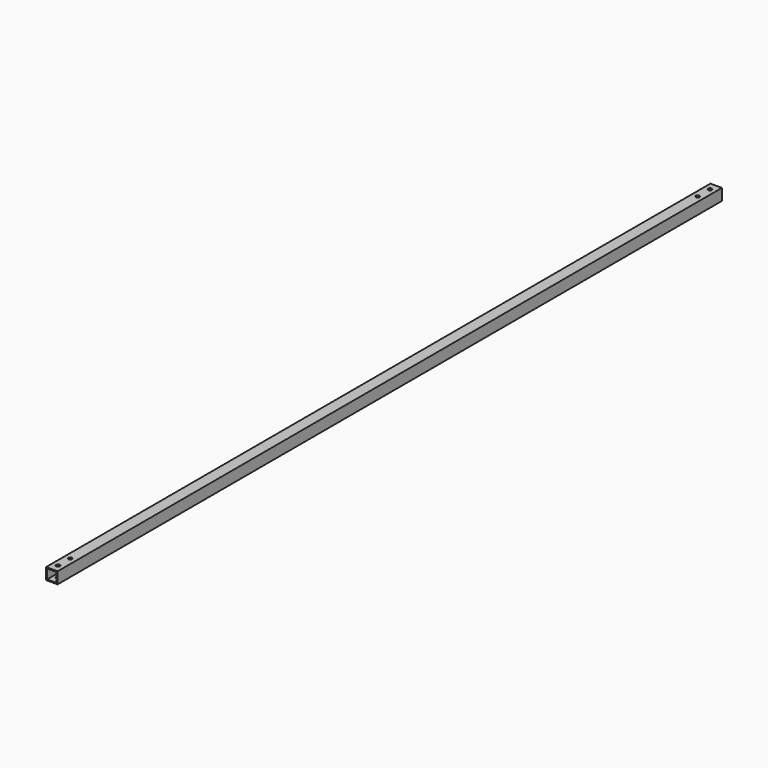
from build123d import *

# Parameters (mm, degrees)
F0_W     = 38.1
F0_H     = 38.1
F0_W_2   = 31.75
F0_H_2   = 31.75
F1_DEPTH = 2743.2
F2_R     = 6.35
F3_DEPTH = 38.101


# Not quite as in the source:
# - a feature names something its author has since deleted; it is built from what else it names


with BuildPart() as f1:
    # F0 (on Front) → F1 (new body)
    with BuildSketch(Plane.XZ):
        Rectangle(F0_W, F0_H)
        Rectangle(F0_W_2, F0_H_2, mode=Mode.SUBTRACT)
    extrude(amount=F1_DEPTH)

    # F2 (on face) → F3 (cut, through all)
    with BuildSketch(Plane.XY.offset(19.05)):
        with Locations((0, -25.4)):
            Circle(F2_R)
        with Locations((0, -76.2)):
            Circle(F2_R)
        with Locations((0, -2717.8)):
            Circle(F2_R)
        with Locations((0, -2667)):
            Circle(F2_R)
    extrude(amount=-F3_DEPTH, mode=Mode.SUBTRACT)


solid = f1.part
